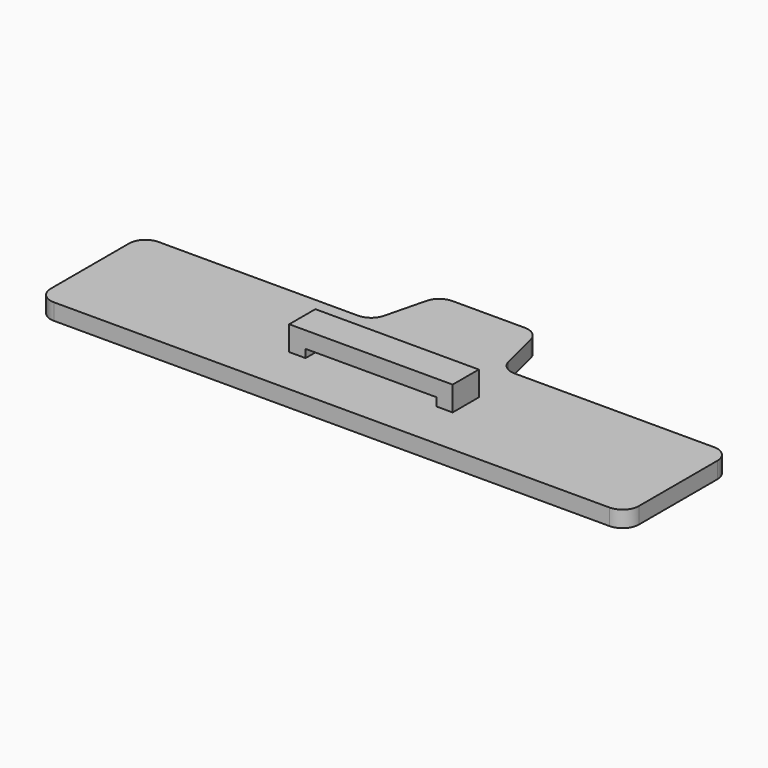
from build123d import *

# Parameters (mm, degrees)
F1_DEPTH = 1.5875
F2_W     = 15.875
F2_H     = 3.175
F3_DEPTH = 2.38125
F5_W     = 12.7
F5_H     = 3.175
F6_DEPTH = 0.79375
F7_R     = 1.5875


# Not quite as in the source:
# - a feature of the source that left no trace in its solid (it failed there, or was rolled back) is left out


with BuildPart() as f1:
    # F0 (on Top) → F1 (new body)
    with BuildSketch(Plane.XY):
        Polygon((28.575, -6.35), (28.575, 6.35), (6.35, 6.35), (4.7625, 12.7), (-4.7625, 12.7), (-6.35, 6.35), (-28.575, 6.35), (-28.575, -6.35), align=None)
    extrude(amount=F1_DEPTH)

    # F2 (on face) → F3 (join)
    with BuildSketch(Plane.XY.offset(1.5875)):
        Rectangle(F2_W, F2_H)
    extrude(amount=F3_DEPTH)

    # F5 (on offset) → F6 (cut)
    with BuildSketch(Plane.XY.offset(2.38125)):
        Rectangle(F5_W, F5_H)
    extrude(amount=-F6_DEPTH, mode=Mode.SUBTRACT)

    # F7
    f7_edges = [f1.edges().sort_by_distance(p)[0] for p in [
        (-28.575, -6.35, 0.79375),
        (28.575, -6.35, 0.79375),
        (28.575, 6.35, 0.79375),
        (4.7625, 12.7, 0.79375),
        (-28.575, 6.35, 0.79375),
        (-4.7625, 12.7, 0.79375),
        (-6.35, 6.35, 0.79375),
        (6.35, 6.35, 0.79375),
    ]]
    fillet(f7_edges, radius=F7_R)


solid = f1.part
